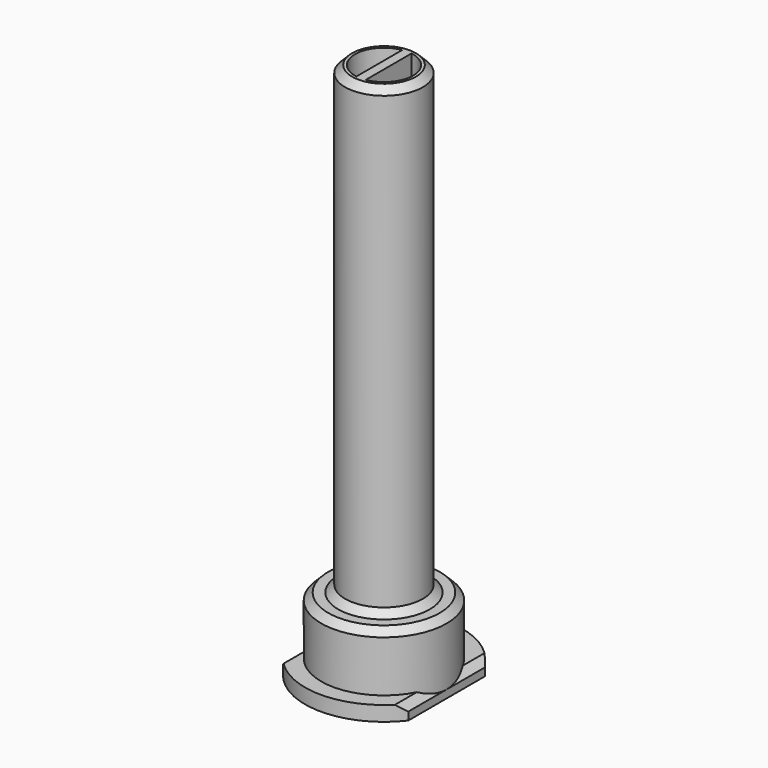
from build123d import *

# Parameters (mm, degrees)
F0_R         = 4.699
F1_DEPTH     = 1.6256
F3_DEPTH     = 3.81
F4_R         = 6.858
F5_DEPTH     = 2.54
F6_R         = 4.25
F7_DEPTH     = 50.8
F8_T8_DEPTH  = 7.2082729301
F8_S9_R      = 6.858
F8_T10_DEPTH = 5
F8_T14_DEPTH = 7.2082729301
F8_S15_R     = 6.858
F8_T16_DEPTH = 5
F8_T22_DEPTH = 7.2082729301
F8_S23_R     = 6.858
F8_T24_DEPTH = 5
F8_T28_DEPTH = 7.2082729301
F8_S29_R     = 6.858
F8_T30_DEPTH = 5


# Not quite as in the source:
# - a fillet or chamfer that OpenCascade refuses, or shapes differently, is made with other operations: its cross-section is extruded or revolved along the edge and cut away or added


with BuildPart() as f1:
    # F0 (on Top) → F1 (new body)
    with BuildSketch(Plane.XY):
        with BuildLine():
            Line((6.858, -5.2486504932), (6.858, 5.2486504932))
            ThreePointArc((6.858, 5.2486504932), (0, 8.636), (-6.858, 5.2486504932))
            Line((-6.858, 5.2486504932), (-6.858, -5.2486504932))
            ThreePointArc((-6.858, -5.2486504932), (0, -8.636), (6.858, -5.2486504932))
        make_face()
        Circle(F0_R, mode=Mode.SUBTRACT)
    extrude(amount=-F1_DEPTH)

    # F2 (on face) → F3 (join)
    with BuildSketch(Plane.XY):
        with BuildLine():
            ThreePointArc((-6.858, 0), (0, -6.858), (6.858, 0))
            ThreePointArc((6.858, 0), (0, 6.858), (-6.858, 0))
        make_face()
        with BuildLine():
            ThreePointArc((0, 3.683), (3.683, 0), (0, -3.683))
            ThreePointArc((0, -3.683), (-3.683, 0), (0, 3.683))
        make_face(mode=Mode.SUBTRACT)
    extrude(amount=F3_DEPTH)

    # F4 (on face) → F5 (join)
    with BuildSketch(Plane.XY.offset(3.81)):
        Circle(F4_R)
        with BuildLine():
            Line((-0.508, 3.1340965205), (-0.508, -3.1340965205))
            ThreePointArc((-0.508, -3.1340965205), (-3.175, 0), (-0.508, 3.1340965205))
        make_face(mode=Mode.SUBTRACT)
        with BuildLine():
            ThreePointArc((0.508, 3.1340965205), (3.175, 0), (0.508, -3.1340965205))
            Line((0.508, -3.1340965205), (0.508, 3.1340965205))
        make_face(mode=Mode.SUBTRACT)
    extrude(amount=F5_DEPTH)

    # F6 (on face) → F7 (join)
    with BuildSketch(Plane.XY.offset(6.35)):
        Circle(F6_R)
        with BuildLine():
            Line((-0.508, 3.1340965205), (-0.508, -3.1340965205))
            ThreePointArc((-0.508, -3.1340965205), (-3.175, 0), (-0.508, 3.1340965205))
        make_face(mode=Mode.SUBTRACT)
        with BuildLine():
            ThreePointArc((0.508, 3.1340965205), (3.175, 0), (0.508, -3.1340965205))
            Line((0.508, -3.1340965205), (0.508, 3.1340965205))
        make_face(mode=Mode.SUBTRACT)
    extrude(amount=F7_DEPTH)

    # F8: chamfer of 0.762 on 5 edges, made by hand

    # F8_s1 → F8_t2 (revolve)
    with BuildSketch(Plane.XZ):
        Polygon((4.25, 7.112), (5.012, 6.35), (4.25, 6.35), align=None)
    revolve(axis=Axis((0, 0, 6.35), (0, 0, 1)))

    # F8_s3 → F8_t4 (revolve, cut)
    with BuildSketch(Plane.XZ):
        Polygon((6.858, 5.588), (6.096, 6.35), (6.858, 6.35), align=None)
    revolve(axis=Axis((0, 0, 6.35), (0, 0, 1)), mode=Mode.SUBTRACT)


with BuildPart() as f8_tool6:
    # F8_s7 → F8_t8 (new body)
    with BuildSketch(Plane.XZ.offset(-7.2082729301)):
        Polygon((-6.096, 0), (-6.858, -0.762), (-6.858, 0), align=None)
    extrude(amount=F8_T8_DEPTH)

    # F8_s9 → F8_t10 (cut, symmetric)
    with BuildSketch(Plane.XY.offset(-0.4)):
        Circle(F8_S9_R)
    extrude(amount=F8_T10_DEPTH, both=True, mode=Mode.SUBTRACT)


with BuildPart() as f1_1:
    add(f1.part)

    # F8_t5: cut F8_tool6
    add(f8_tool6.part, mode=Mode.SUBTRACT)


with BuildPart() as f8_tool12:
    # F8_s13 → F8_t14 (new body)
    with BuildSketch(Plane.XZ):
        Polygon((6.858, -0.762), (6.096, 0), (6.858, 0), align=None)
    extrude(amount=-F8_T14_DEPTH)

    # F8_s15 → F8_t16 (cut, symmetric)
    with BuildSketch(Plane.XY.offset(-0.4)):
        Circle(F8_S15_R)
    extrude(amount=F8_T16_DEPTH, both=True, mode=Mode.SUBTRACT)


with BuildPart() as f1_2:
    add(f1_1.part)

    # F8_t11: cut F8_tool12
    add(f8_tool12.part, mode=Mode.SUBTRACT)

    # F8_s17 → F8_t18 (revolve, cut)
    with BuildSketch(Plane.XZ):
        Polygon((4.25, 56.388), (3.488, 57.15), (4.25, 57.15), align=None)
    revolve(axis=Axis((0, 0, 57.15), (0, 0, 1)), mode=Mode.SUBTRACT)


with BuildPart() as f8_tool20:
    # F8_s21 → F8_t22 (new body)
    with BuildSketch(Plane.XZ.offset(7.2082729301)):
        Polygon((6.858, -0.762), (6.096, 0), (6.858, 0), align=None)
    extrude(amount=-F8_T22_DEPTH)

    # F8_s23 → F8_t24 (cut, symmetric)
    with BuildSketch(Plane.XY.offset(-0.4)):
        Circle(F8_S23_R)
    extrude(amount=F8_T24_DEPTH, both=True, mode=Mode.SUBTRACT)


with BuildPart() as f1_3:
    add(f1_2.part)

    # F8_t19: cut F8_tool20
    add(f8_tool20.part, mode=Mode.SUBTRACT)


with BuildPart() as f8_tool26:
    # F8_s27 → F8_t28 (new body)
    with BuildSketch(Plane.XZ):
        Polygon((-6.096, 0), (-6.858, -0.762), (-6.858, 0), align=None)
    extrude(amount=F8_T28_DEPTH)

    # F8_s29 → F8_t30 (cut, symmetric)
    with BuildSketch(Plane.XY.offset(-0.4)):
        Circle(F8_S29_R)
    extrude(amount=F8_T30_DEPTH, both=True, mode=Mode.SUBTRACT)


with BuildPart() as f1_4:
    add(f1_3.part)

    # F8_t25: cut F8_tool26
    add(f8_tool26.part, mode=Mode.SUBTRACT)


solid = f1_4.part
